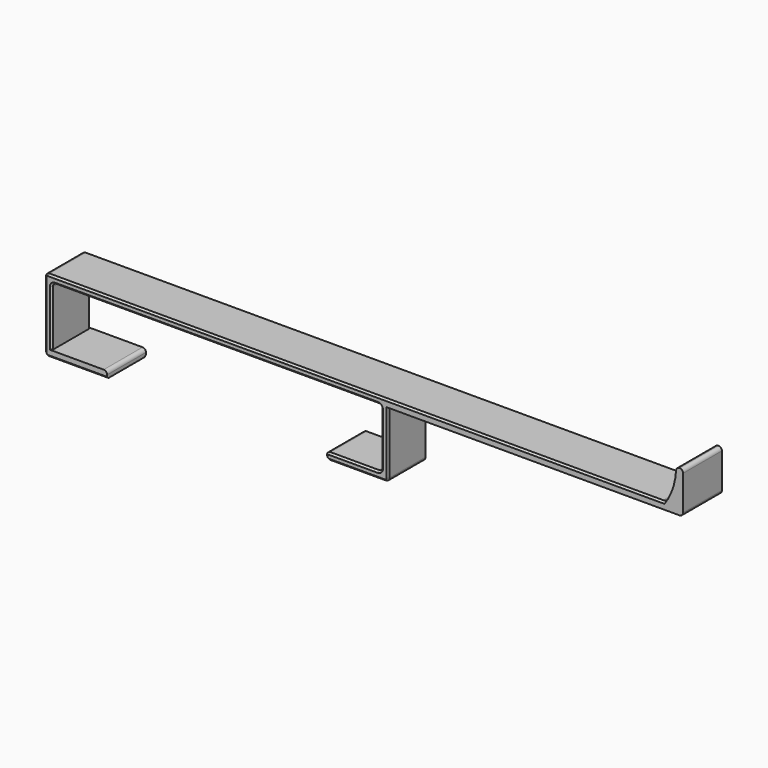
from build123d import *

# Parameters (mm, degrees)
F1_DEPTH = 14
F2_R     = 0.99999
F3_SIZE  = 0.5
F4_R     = 2


# Not quite as in the source:
# - a fillet or chamfer is up to 0.001 mm smaller than in the source, because OpenCascade refuses the exact size


with BuildPart() as f1:
    # F0 (on Front) → F1 (new body)
    with BuildSketch(Plane.XZ):
        with BuildLine():
            Line((-68.4901475161, 21), (-167.4901475161, 21))
            Line((-167.4901475161, 21), (-167.4901475161, 0))
            Line((-167.4901475161, 0), (-149.4901475161, 0))
            Line((-149.4901475161, 0), (-149.4901475161, 2))
            Line((-149.4901475161, 2), (-165.4901475161, 2))
            Line((-165.4901475161, 2), (-165.4901475161, 19))
            Line((-165.4901475161, 19), (-70.4901475161, 19))
            Line((-70.4901475161, 19), (-70.4901475161, 2))
            Line((-70.4901475161, 2), (-86.4901475161, 2))
            Line((-86.4901475161, 2), (-86.4901475161, 0))
            Line((-86.4901475161, 0), (-68.4901475161, 0))
            Line((-68.4901475161, 0), (-68.4901475161, 19))
            Line((-68.4901475161, 19), (16.5098524839, 19))
            Line((16.5098524839, 19), (16.5098524839, 21))
            Line((16.5098524839, 21), (16.5098524839, 31))
            Line((16.5098524839, 31), (14.5098524839, 31))
            ThreePointArc((14.5098524839, 31), (13.7436966654, 25.7798467455), (11.5098524839, 21))
            Line((11.5098524839, 21), (-63.147776881, 21))
            Line((-63.147776881, 21), (-68.4901475161, 21))
        make_face()
    extrude(amount=F1_DEPTH)

    # F2 (radius 1 in the source; OpenCascade refuses exactly that, so slightly less here)
    f2_edges = [f1.edges().sort_by_distance(p)[0] for p in [
        (14.509852, -7, 31),
        (16.509852, -7, 31),
        (16.509852, -7, 19),
        (-70.490148, -7, 2),
        (-70.490148, -7, 19),
        (-86.490148, -7, 2),
        (-86.490148, -7, 0),
        (-68.490148, -7, 0),
        (-165.490148, -7, 19),
        (-149.490148, -7, 2),
        (-167.490148, -7, 0),
        (-167.490148, -7, 21),
    ]]
    fillet(f2_edges, radius=F2_R)

    # F3
    f3_edges = [f1.edges().sort_by_distance(p)[0] for p in [
        (-77.490153, 0, 21),
        (-117.990148, 0, 19),
        (-167.490148, -14, 10.5),
        (-68.490148, -14, 9.999995),
    ]]
    chamfer(f3_edges, length=F3_SIZE)

    # F4
    f4_edges = [f1.edges().sort_by_distance(p)[0] for p in [
        (11.509852, -7, 21),
    ]]
    fillet(f4_edges, radius=F4_R)


solid = f1.part
